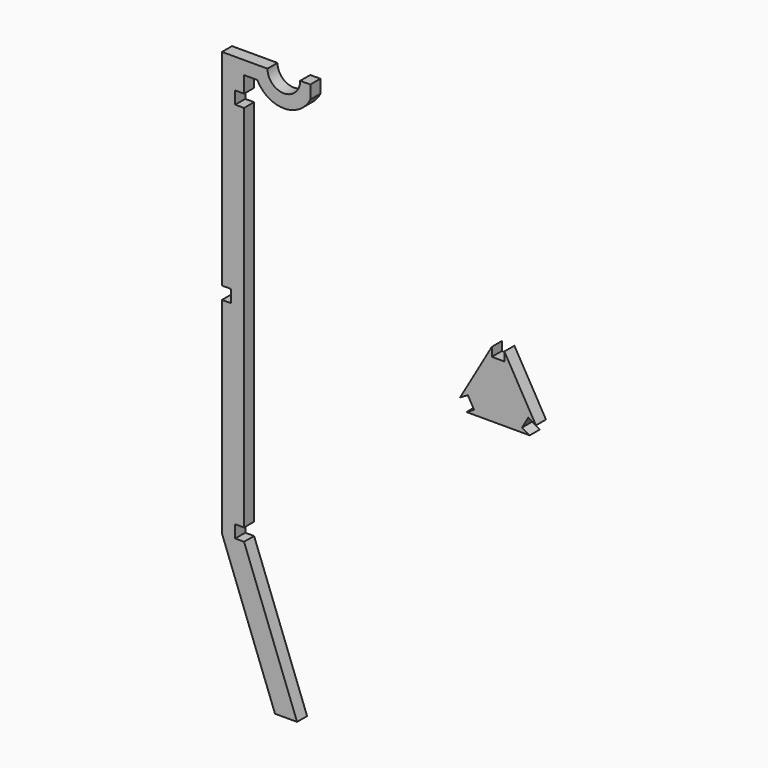
from build123d import *

# Parameters (mm, degrees)
F1_W     = 19.05
F1_H     = 19.05
F2_DEPTH = 18.034


# Not quite as in the source:
# - a variable given as a bare number and used for a length is read in inches; the dataset says mm whatever the document's units were


with BuildPart() as f2:
    # F1 (on Front) → F2 (new body)
    with BuildSketch(Plane.XZ):
        Polygon((15.875, 285.75), (15.875, 304.8), (-15.875, 304.8), (-15.875, 9.017), (-3.175, 9.017), (-3.175, 0), (-3.175, -9.017), (-15.875, -9.017), (-15.875, -304.8), (3.175, -304.8), (3.175, -286.766), (15.875, -286.766), (15.875, 244.1689050286), (3.175, 244.1689050286), (3.175, 262.2029050286), (15.875, 262.2029050286), align=None)
        with BuildLine():
            Line((49.4779050286, 304.8), (34.925, 304.8))
            Line((34.925, 304.8), (34.925, 285.75))
            ThreePointArc((34.925, 285.75), (73.025, 262.2029050286), (111.125, 285.75))
            Line((111.125, 285.75), (111.125, 304.8))
            Line((111.125, 304.8), (96.5720949714, 304.8))
            ThreePointArc((96.5720949714, 304.8), (73.025, 281.2529050286), (49.4779050286, 304.8))
        make_face()
        with Locations((25.4, 295.275)):
            Rectangle(F1_W, F1_H)
        Polygon((3.175, -304.8), (-15.875, -304.8), (60.325, -508), (92.075, -508), (15.875, -304.8), align=None)
    extrude(amount=F2_DEPTH)


with BuildPart() as f2b:
    # F1 (on Front) → F2, piece 2 (new body)
    with BuildSketch(Plane.XZ):
        Polygon((435.483, -21.0438399617), (390.017, 57.7055820552), (390.017, 45.0055820552), (371.983, 45.0055820552), (371.983, 57.7055820552), (326.517, -21.0438399617), (337.5155226281, -14.6938399617), (346.5325226281, -30.3117420935), (335.534, -36.6617420935), (426.466, -36.6617420935), (415.4674773719, -30.3117420935), (424.4844773719, -14.6938399617), align=None)
    extrude(amount=F2_DEPTH)


solid = Compound([f2.part, f2b.part])
